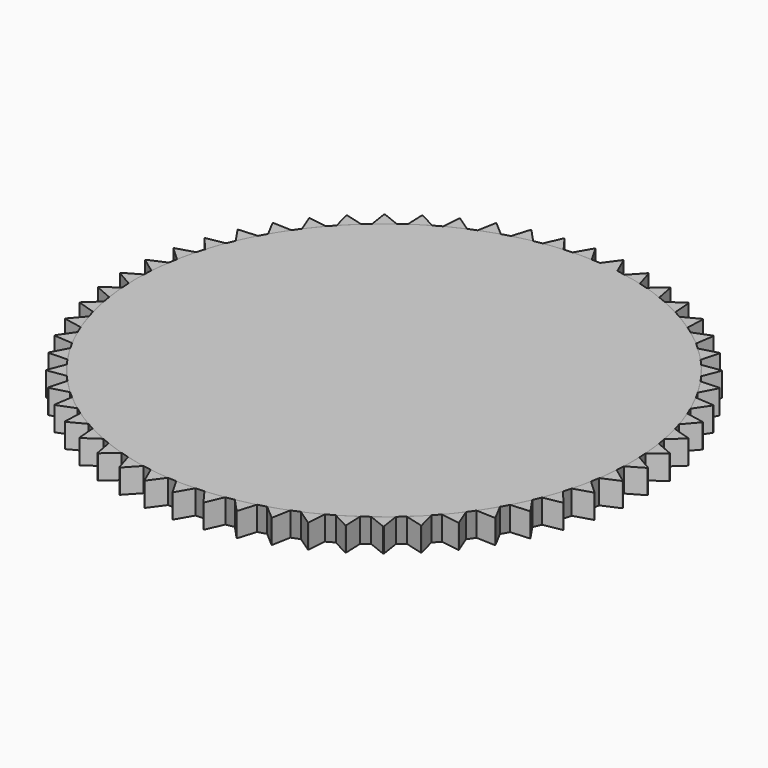
from build123d import *

# Parameters (mm, degrees)
F1_DEPTH = 1.27
F2_R     = 0.0254
F4_COUNT = 56


with BuildPart() as f1:
    # F0 (on Top) → F1 (new body)
    with BuildSketch(Plane.XY):
        with BuildLine():
            Line((0, 13.97), (-0.508, 13.0870191704))
            ThreePointArc((-0.508, 13.0870191704), (0, -13.096875), (0.508, 13.0870191704))
            Line((0.508, 13.0870191704), (0, 13.97))
        make_face()
    extrude(amount=F1_DEPTH)

    # F2
    f2_edges = [f1.edges().sort_by_distance(p)[0] for p in [
        (0, 13.97, 0.635),
    ]]
    fillet(f2_edges, radius=F2_R)


with BuildPart() as f4_1:
    # F4: instance of F1
    add(f1.part.rotate(Axis((0, 0, 6.4253821038), (0, 0, 1)), 1 * 360 / F4_COUNT))


with BuildPart() as f4_2:
    # F4: instance of F1
    add(f1.part.rotate(Axis((0, 0, 6.4253821038), (0, 0, 1)), 2 * 360 / F4_COUNT))


with BuildPart() as f4_3:
    # F4: instance of F1
    add(f1.part.rotate(Axis((0, 0, 6.4253821038), (0, 0, 1)), 3 * 360 / F4_COUNT))


with BuildPart() as f4_4:
    # F4: instance of F1
    add(f1.part.rotate(Axis((0, 0, 6.4253821038), (0, 0, 1)), 4 * 360 / F4_COUNT))


with BuildPart() as f4_5:
    # F4: instance of F1
    add(f1.part.rotate(Axis((0, 0, 6.4253821038), (0, 0, 1)), 5 * 360 / F4_COUNT))


with BuildPart() as f4_6:
    # F4: instance of F1
    add(f1.part.rotate(Axis((0, 0, 6.4253821038), (0, 0, 1)), 6 * 360 / F4_COUNT))


with BuildPart() as f4_7:
    # F4: instance of F1
    add(f1.part.rotate(Axis((0, 0, 6.4253821038), (0, 0, 1)), 7 * 360 / F4_COUNT))


with BuildPart() as f4_8:
    # F4: instance of F1
    add(f1.part.rotate(Axis((0, 0, 6.4253821038), (0, 0, 1)), 8 * 360 / F4_COUNT))


with BuildPart() as f4_9:
    # F4: instance of F1
    add(f1.part.rotate(Axis((0, 0, 6.4253821038), (0, 0, 1)), 9 * 360 / F4_COUNT))


with BuildPart() as f4_10:
    # F4: instance of F1
    add(f1.part.rotate(Axis((0, 0, 6.4253821038), (0, 0, 1)), 10 * 360 / F4_COUNT))


with BuildPart() as f4_11:
    # F4: instance of F1
    add(f1.part.rotate(Axis((0, 0, 6.4253821038), (0, 0, 1)), 11 * 360 / F4_COUNT))


with BuildPart() as f4_12:
    # F4: instance of F1
    add(f1.part.rotate(Axis((0, 0, 6.4253821038), (0, 0, 1)), 12 * 360 / F4_COUNT))


with BuildPart() as f4_13:
    # F4: instance of F1
    add(f1.part.rotate(Axis((0, 0, 6.4253821038), (0, 0, 1)), 13 * 360 / F4_COUNT))


with BuildPart() as f4_14:
    # F4: instance of F1
    add(f1.part.rotate(Axis((0, 0, 6.4253821038), (0, 0, 1)), 14 * 360 / F4_COUNT))


with BuildPart() as f4_15:
    # F4: instance of F1
    add(f1.part.rotate(Axis((0, 0, 6.4253821038), (0, 0, 1)), 15 * 360 / F4_COUNT))


with BuildPart() as f4_16:
    # F4: instance of F1
    add(f1.part.rotate(Axis((0, 0, 6.4253821038), (0, 0, 1)), 16 * 360 / F4_COUNT))


with BuildPart() as f4_17:
    # F4: instance of F1
    add(f1.part.rotate(Axis((0, 0, 6.4253821038), (0, 0, 1)), 17 * 360 / F4_COUNT))


with BuildPart() as f4_18:
    # F4: instance of F1
    add(f1.part.rotate(Axis((0, 0, 6.4253821038), (0, 0, 1)), 18 * 360 / F4_COUNT))


with BuildPart() as f4_19:
    # F4: instance of F1
    add(f1.part.rotate(Axis((0, 0, 6.4253821038), (0, 0, 1)), 19 * 360 / F4_COUNT))


with BuildPart() as f4_20:
    # F4: instance of F1
    add(f1.part.rotate(Axis((0, 0, 6.4253821038), (0, 0, 1)), 20 * 360 / F4_COUNT))


with BuildPart() as f4_21:
    # F4: instance of F1
    add(f1.part.rotate(Axis((0, 0, 6.4253821038), (0, 0, 1)), 21 * 360 / F4_COUNT))


with BuildPart() as f4_22:
    # F4: instance of F1
    add(f1.part.rotate(Axis((0, 0, 6.4253821038), (0, 0, 1)), 22 * 360 / F4_COUNT))


with BuildPart() as f4_23:
    # F4: instance of F1
    add(f1.part.rotate(Axis((0, 0, 6.4253821038), (0, 0, 1)), 23 * 360 / F4_COUNT))


with BuildPart() as f4_24:
    # F4: instance of F1
    add(f1.part.rotate(Axis((0, 0, 6.4253821038), (0, 0, 1)), 24 * 360 / F4_COUNT))


with BuildPart() as f4_25:
    # F4: instance of F1
    add(f1.part.rotate(Axis((0, 0, 6.4253821038), (0, 0, 1)), 25 * 360 / F4_COUNT))


with BuildPart() as f4_26:
    # F4: instance of F1
    add(f1.part.rotate(Axis((0, 0, 6.4253821038), (0, 0, 1)), 26 * 360 / F4_COUNT))


with BuildPart() as f4_27:
    # F4: instance of F1
    add(f1.part.rotate(Axis((0, 0, 6.4253821038), (0, 0, 1)), 27 * 360 / F4_COUNT))


with BuildPart() as f4_28:
    # F4: instance of F1
    add(f1.part.rotate(Axis((0, 0, 6.4253821038), (0, 0, 1)), 28 * 360 / F4_COUNT))


with BuildPart() as f4_29:
    # F4: instance of F1
    add(f1.part.rotate(Axis((0, 0, 6.4253821038), (0, 0, 1)), 29 * 360 / F4_COUNT))


with BuildPart() as f4_30:
    # F4: instance of F1
    add(f1.part.rotate(Axis((0, 0, 6.4253821038), (0, 0, 1)), 30 * 360 / F4_COUNT))


with BuildPart() as f4_31:
    # F4: instance of F1
    add(f1.part.rotate(Axis((0, 0, 6.4253821038), (0, 0, 1)), 31 * 360 / F4_COUNT))


with BuildPart() as f4_32:
    # F4: instance of F1
    add(f1.part.rotate(Axis((0, 0, 6.4253821038), (0, 0, 1)), 32 * 360 / F4_COUNT))


with BuildPart() as f4_33:
    # F4: instance of F1
    add(f1.part.rotate(Axis((0, 0, 6.4253821038), (0, 0, 1)), 33 * 360 / F4_COUNT))


with BuildPart() as f4_34:
    # F4: instance of F1
    add(f1.part.rotate(Axis((0, 0, 6.4253821038), (0, 0, 1)), 34 * 360 / F4_COUNT))


with BuildPart() as f4_35:
    # F4: instance of F1
    add(f1.part.rotate(Axis((0, 0, 6.4253821038), (0, 0, 1)), 35 * 360 / F4_COUNT))


with BuildPart() as f4_36:
    # F4: instance of F1
    add(f1.part.rotate(Axis((0, 0, 6.4253821038), (0, 0, 1)), 36 * 360 / F4_COUNT))


with BuildPart() as f4_37:
    # F4: instance of F1
    add(f1.part.rotate(Axis((0, 0, 6.4253821038), (0, 0, 1)), 37 * 360 / F4_COUNT))


with BuildPart() as f4_38:
    # F4: instance of F1
    add(f1.part.rotate(Axis((0, 0, 6.4253821038), (0, 0, 1)), 38 * 360 / F4_COUNT))


with BuildPart() as f4_39:
    # F4: instance of F1
    add(f1.part.rotate(Axis((0, 0, 6.4253821038), (0, 0, 1)), 39 * 360 / F4_COUNT))


with BuildPart() as f4_40:
    # F4: instance of F1
    add(f1.part.rotate(Axis((0, 0, 6.4253821038), (0, 0, 1)), 40 * 360 / F4_COUNT))


with BuildPart() as f4_41:
    # F4: instance of F1
    add(f1.part.rotate(Axis((0, 0, 6.4253821038), (0, 0, 1)), 41 * 360 / F4_COUNT))


with BuildPart() as f4_42:
    # F4: instance of F1
    add(f1.part.rotate(Axis((0, 0, 6.4253821038), (0, 0, 1)), 42 * 360 / F4_COUNT))


with BuildPart() as f4_43:
    # F4: instance of F1
    add(f1.part.rotate(Axis((0, 0, 6.4253821038), (0, 0, 1)), 43 * 360 / F4_COUNT))


with BuildPart() as f4_44:
    # F4: instance of F1
    add(f1.part.rotate(Axis((0, 0, 6.4253821038), (0, 0, 1)), 44 * 360 / F4_COUNT))


with BuildPart() as f4_45:
    # F4: instance of F1
    add(f1.part.rotate(Axis((0, 0, 6.4253821038), (0, 0, 1)), 45 * 360 / F4_COUNT))


with BuildPart() as f4_46:
    # F4: instance of F1
    add(f1.part.rotate(Axis((0, 0, 6.4253821038), (0, 0, 1)), 46 * 360 / F4_COUNT))


with BuildPart() as f4_47:
    # F4: instance of F1
    add(f1.part.rotate(Axis((0, 0, 6.4253821038), (0, 0, 1)), 47 * 360 / F4_COUNT))


with BuildPart() as f4_48:
    # F4: instance of F1
    add(f1.part.rotate(Axis((0, 0, 6.4253821038), (0, 0, 1)), 48 * 360 / F4_COUNT))


with BuildPart() as f4_49:
    # F4: instance of F1
    add(f1.part.rotate(Axis((0, 0, 6.4253821038), (0, 0, 1)), 49 * 360 / F4_COUNT))


with BuildPart() as f4_50:
    # F4: instance of F1
    add(f1.part.rotate(Axis((0, 0, 6.4253821038), (0, 0, 1)), 50 * 360 / F4_COUNT))


with BuildPart() as f4_51:
    # F4: instance of F1
    add(f1.part.rotate(Axis((0, 0, 6.4253821038), (0, 0, 1)), 51 * 360 / F4_COUNT))


with BuildPart() as f4_52:
    # F4: instance of F1
    add(f1.part.rotate(Axis((0, 0, 6.4253821038), (0, 0, 1)), 52 * 360 / F4_COUNT))


with BuildPart() as f4_53:
    # F4: instance of F1
    add(f1.part.rotate(Axis((0, 0, 6.4253821038), (0, 0, 1)), 53 * 360 / F4_COUNT))


with BuildPart() as f4_54:
    # F4: instance of F1
    add(f1.part.rotate(Axis((0, 0, 6.4253821038), (0, 0, 1)), 54 * 360 / F4_COUNT))


with BuildPart() as f4_55:
    # F4: instance of F1
    add(f1.part.rotate(Axis((0, 0, 6.4253821038), (0, 0, 1)), 55 * 360 / F4_COUNT))


solid = Compound([f1.part, f4_1.part, f4_2.part, f4_3.part, f4_4.part, f4_5.part, f4_6.part, f4_7.part, f4_8.part, f4_9.part, f4_10.part, f4_11.part, f4_12.part, f4_13.part, f4_14.part, f4_15.part, f4_16.part, f4_17.part, f4_18.part, f4_19.part, f4_20.part, f4_21.part, f4_22.part, f4_23.part, f4_24.part, f4_25.part, f4_26.part, f4_27.part, f4_28.part, f4_29.part, f4_30.part, f4_31.part, f4_32.part, f4_33.part, f4_34.part, f4_35.part, f4_36.part, f4_37.part, f4_38.part, f4_39.part, f4_40.part, f4_41.part, f4_42.part, f4_43.part, f4_44.part, f4_45.part, f4_46.part, f4_47.part, f4_48.part, f4_49.part, f4_50.part, f4_51.part, f4_52.part, f4_53.part, f4_54.part, f4_55.part])
